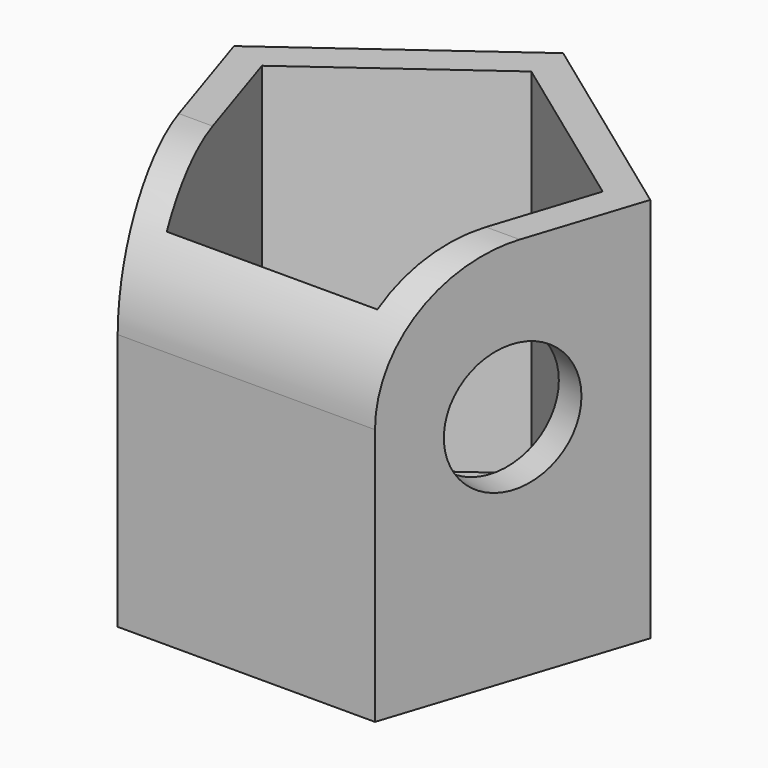
from build123d import *

# Parameters (mm, degrees)
F1_DEPTH    = 30
F2_T        = -2.5
F3_R        = 5
F4_DEPTH    = 12.6
F5_T1_DEPTH = 70


# Not quite as in the source:
# - a fillet or chamfer that OpenCascade refuses, or shapes differently, is made with other operations: its cross-section is extruded or revolved along the edge and cut away or added


with BuildPart() as f1:
    # F0 (on Top) → F1 (new body)
    with BuildSketch(Plane.XY):
        Polygon((16.1803398875, 5.2573111212), (0, 17.013016167), (-16.1803398875, 5.2573111212), (-10, -13.7638192047), (10, -13.7638192047), align=None)
    extrude(amount=F1_DEPTH)

    # F2
    f2_openings = [f1.faces().sort_by_distance(p)[0] for p in [
        (0, 0, 30),
    ]]
    offset(amount=F2_T, openings=f2_openings)

    # F3 (on face) → F4 (cut)
    with BuildSketch(Plane(origin=(13.0901699437, -4.2532540418, 0), x_dir=(0.3090169944, 0.9510565163, 0), z_dir=(0.9510565163, -0.3090169944, 0))):
        with Locations((0, 18)):
            Circle(F3_R)
    extrude(amount=-F4_DEPTH, mode=Mode.SUBTRACT)

    # F5: fillet of radius 10 on 1 edges, made by hand

    # F5_s2 → F5_t1 (cut)
    with BuildSketch(Plane.YZ.offset(-35)):
        with BuildLine():
            ThreePointArc((-3.7638192047, 30), (-10.8348870166, 27.0710678119), (-13.7638192047, 20))
            Line((-13.7638192047, 20), (-13.7638192047, 30))
            Line((-13.7638192047, 30), (-3.7638192047, 30))
        make_face()
    extrude(amount=F5_T1_DEPTH, mode=Mode.SUBTRACT)


solid = f1.part
